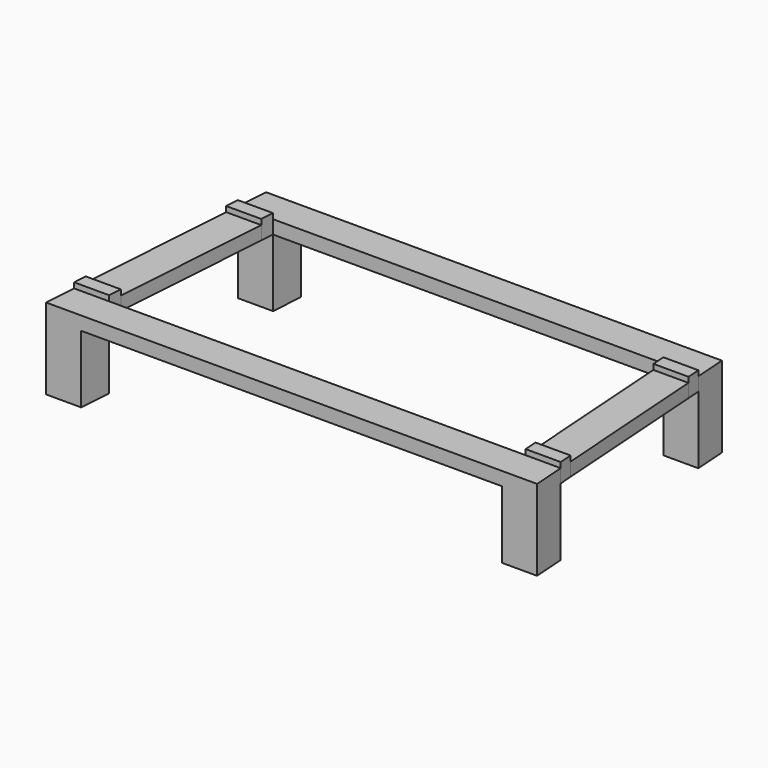
from build123d import *

# Parameters (mm, degrees)
F1_DEPTH = 30
F2_DEPTH = 5
F3_DEPTH = 2


with BuildPart() as f1:
    # F0 (on Top) → F1 (new body)
    with BuildSketch(Plane.XY):
        Polygon((-84.5, 46.8874983338), (-85.329787234, 34.9162221635), (-72.329787234, 34.9162221635), (-71.5, 46.8874983338), align=None)
    extrude(amount=-F1_DEPTH)



with BuildPart() as f1b:
    # F0 (on Top) → F1, piece 2 (new body)
    with BuildSketch(Plane.XY):
        Polygon((71.5, 46.8874983338), (72.329787234, 34.9162221635), (85.329787234, 34.9162221635), (84.5, 46.8874983338), align=None)
    extrude(amount=-F1_DEPTH)


with BuildPart() as f1c:
    # F0 (on Top) → F1, piece 3 (new body)
    with BuildSketch(Plane.XY):
        Polygon((77.170212766, -34.9162221635), (78, -46.8874983338), (91, -46.8874983338), (90.170212766, -34.9162221635), align=None)
    extrude(amount=-F1_DEPTH)


with BuildPart() as f1d:
    # F0 (on Top) → F1, piece 4 (new body)
    with BuildSketch(Plane.XY):
        Polygon((-90.170212766, -34.9162221635), (-91, -46.8874983338), (-78, -46.8874983338), (-77.170212766, -34.9162221635), align=None)
    extrude(amount=-F1_DEPTH)


with BuildPart() as f1_1:
    add(f1.part)

    add(f1b.part)  # F2 merges F1b

    add(f1c.part)  # F2 merges F1c

    add(f1d.part)  # F2 merges F1d
    # F0 (on Top) → F2 (join)
    with BuildSketch(Plane.XY):
        Polygon((-85.6763614932, 29.9162221635), (-89.8236385068, -29.9162221635), (-76.8236385068, -29.9162221635), (-72.6763614932, 29.9162221635), align=None)
        Polygon((-85.329787234, 34.9162221635), (-85.6763614932, 29.9162221635), (-72.6763614932, 29.9162221635), (-72.329787234, 34.9162221635), align=None)
        Polygon((-89.8236385068, -29.9162221635), (-90.170212766, -34.9162221635), (-77.170212766, -34.9162221635), (-76.8236385068, -29.9162221635), align=None)
        Polygon((-77.170212766, -34.9162221635), (-78, -46.8874983338), (-72.988003021, -46.8874983338), (-72.158215787, -34.9162221635), align=None)
        Polygon((-72.158215787, -34.9162221635), (-72.988003021, -46.8874983338), (72.988003021, -46.8874983338), (72.158215787, -34.9162221635), align=None)
        Polygon((72.158215787, -34.9162221635), (72.988003021, -46.8874983338), (78, -46.8874983338), (77.170212766, -34.9162221635), align=None)
        Polygon((76.8236385068, -29.9162221635), (77.170212766, -34.9162221635), (90.170212766, -34.9162221635), (89.8236385068, -29.9162221635), align=None)
        Polygon((72.6763614932, 29.9162221635), (76.8236385068, -29.9162221635), (89.8236385068, -29.9162221635), (85.6763614932, 29.9162221635), align=None)
        Polygon((72.329787234, 34.9162221635), (72.6763614932, 29.9162221635), (85.6763614932, 29.9162221635), (85.329787234, 34.9162221635), align=None)
        Polygon((66.488003021, 46.8874983338), (67.3177902551, 34.9162221635), (72.329787234, 34.9162221635), (71.5, 46.8874983338), align=None)
        Polygon((-66.488003021, 46.8874983338), (-67.3177902551, 34.9162221635), (67.3177902551, 34.9162221635), (66.488003021, 46.8874983338), align=None)
        Polygon((-71.5, 46.8874983338), (-72.329787234, 34.9162221635), (-67.3177902551, 34.9162221635), (-66.488003021, 46.8874983338), align=None)
    extrude(amount=-F2_DEPTH)

    # F0 (on Top) → F3 (join)
    with BuildSketch(Plane.XY):
        Polygon((-85.329787234, 34.9162221635), (-85.6763614932, 29.9162221635), (-72.6763614932, 29.9162221635), (-72.329787234, 34.9162221635), align=None)
        Polygon((-89.8236385068, -29.9162221635), (-90.170212766, -34.9162221635), (-77.170212766, -34.9162221635), (-76.8236385068, -29.9162221635), align=None)
        Polygon((72.329787234, 34.9162221635), (72.6763614932, 29.9162221635), (85.6763614932, 29.9162221635), (85.329787234, 34.9162221635), align=None)
        Polygon((76.8236385068, -29.9162221635), (77.170212766, -34.9162221635), (90.170212766, -34.9162221635), (89.8236385068, -29.9162221635), align=None)
    extrude(amount=F3_DEPTH)


solid = f1_1.part
